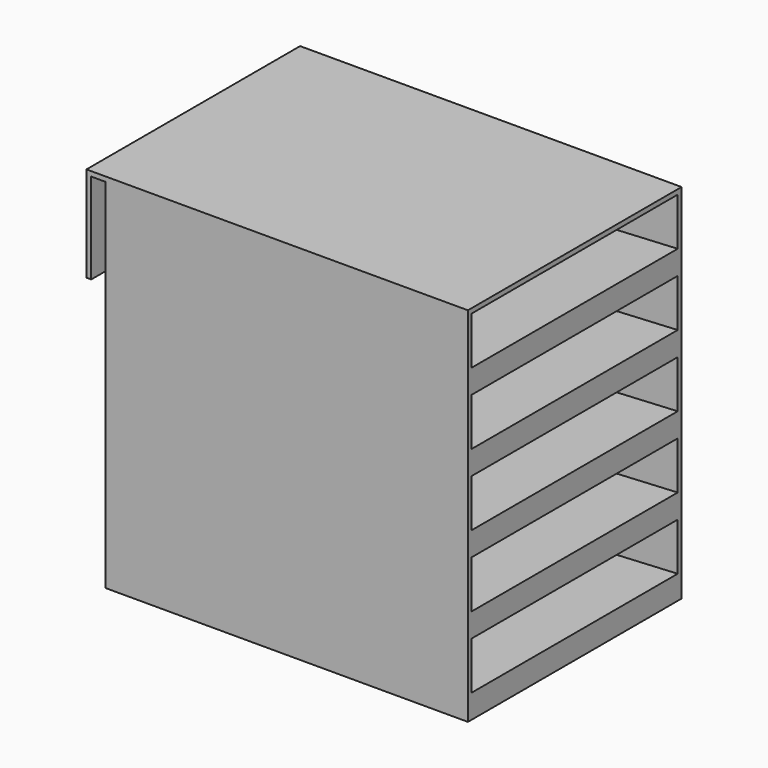
from build123d import *

# Parameters (mm, degrees)
F0_W           = 76
F0_H           = 76
F1_DEPTH       = 28
F2_W           = 54
F2_H           = 10
F5_W           = 56
F5_H           = 76
F6_DEPTH       = 1
F8_DEPTH       = 56
F9_TEXT_SIZE   = 8.9253324808
F9_TEXT_SIZE_2 = 9.2617753479
F9_TEXT_SIZE_3 = 9.3902593815
F9_TEXT_SIZE_4 = 9.6482923254
F9_TEXT_SIZE_5 = 10.8240379228
F10_DEPTH      = 1


# Not quite as in the source:
# - Text() gives the source's letters only with a copy of the font that has no kerning and outlines rounded to 1/6400 em; it was checked with that copy


with BuildPart() as f1:
    # F0 (on Front) → F1 (new body, symmetric)
    with BuildSketch(Plane.XZ):
        Rectangle(F0_W, F0_H)
    extrude(amount=F1_DEPTH, both=True)

    # F4: sweep along a path in F3
    with BuildLine(Plane.XZ.offset(28)) as f4_path:
        Line((38, 37), (-38, 33.0170087745))
    # F2 (on face) → F4 (sweep, cut)
    with BuildSketch(Plane.YZ.offset(38)):
        with Locations((0, 32)):
            Rectangle(F2_W, F2_H)
        with Locations((0, 17)):
            Rectangle(F2_W, F2_H)
        with Locations((0, 2)):
            Rectangle(F2_W, F2_H)
        with Locations((0, -13)):
            Rectangle(F2_W, F2_H)
        with Locations((0, -28)):
            Rectangle(F2_W, F2_H)
    sweep(path=f4_path.line, mode=Mode.SUBTRACT)

    # F5 (on face) → F6 (join)
    with BuildSketch(Plane(origin=(-38, 0, 0), x_dir=(0, -1, 0), z_dir=(-1, 0, 0))):
        Rectangle(F5_W, F5_H)
    extrude(amount=-F6_DEPTH)

    # F7 (on face) → F8 (join)
    with BuildSketch(Plane.XZ.offset(28)):
        Polygon((-38, 37), (-38, 38), (-42, 38), (-42, 18), (-41, 18), (-41, 37), align=None)
    extrude(amount=-F8_DEPTH)

    # F9 (on face) → F10 (join)
    with BuildSketch(Plane(origin=(0, 28, 0), x_dir=(-1, 0, 0), z_dir=(0, 1, 0))):
        with Locations((-30.6668113917, 28.5186786205)):
            Text('A', F9_TEXT_SIZE, font='Open Sans', text_align=(TextAlign.LEFT, TextAlign.BOTTOM))
        with Locations((-30.4371416569, 12.921391055)):
            Text('B', F9_TEXT_SIZE_2, font='Open Sans', text_align=(TextAlign.LEFT, TextAlign.BOTTOM))
        with Locations((-29.9739278853, -1.6359465662)):
            Text('C', F9_TEXT_SIZE_3, font='Open Sans', text_align=(TextAlign.LEFT, TextAlign.BOTTOM))
        with Locations((-29.9739278853, -16.6555196047)):
            Text('D', F9_TEXT_SIZE_4, font='Open Sans', text_align=(TextAlign.LEFT, TextAlign.BOTTOM))
        with Locations((-29.9739278853, -33.0321379006)):
            Text('E', F9_TEXT_SIZE_5, font='Open Sans', text_align=(TextAlign.LEFT, TextAlign.BOTTOM))
    extrude(amount=F10_DEPTH)


solid = f1.part
